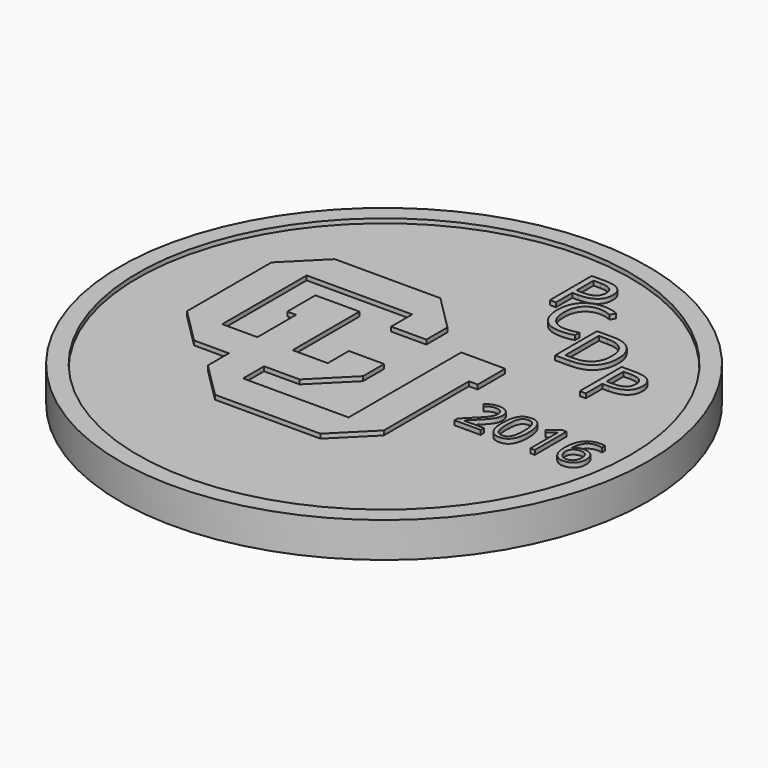
from build123d import *

# Parameters (mm, degrees)
F0_R           = 38.1
F1_DEPTH       = 3.81
F2_R           = 38.1
F2_R_2         = 35.56
F2_TEXT_SIZE   = 10.5833333333
F2_TEXT_SIZE_2 = 8.024699837
F3_DEPTH       = 0.635
F4_R           = 38.1
F4_R_2         = 35.56
F4_TEXT_SIZE   = 14.9135865892
F4_TEXT_SIZE_2 = 16.7777839427
F5_DEPTH       = 0.635


# Not quite as in the source:
# - Text() gives the source's letters only with a copy of the font that has no kerning and outlines rounded to 1/6400 em; it was checked with that copy


with BuildPart() as f1:
    # F0 (on Top) → F1 (new body)
    with BuildSketch(Plane.XY):
        Circle(F0_R)
    extrude(amount=F1_DEPTH)

    # F2 (on face) → F3 (join)
    with BuildSketch(Plane.XY.offset(3.81)):
        Circle(F2_R)
        Circle(F2_R_2, mode=Mode.SUBTRACT)
        Polygon((0, -3.81), (0, 0), (-5.08, 0), (-5.08, -3.81), (-10.16, -3.81), (-10.16, 8.252271885), (-16.51, 8.252271885), (-16.51, 3.172271885), (-15.24, 3.172271885), (-15.24, -3.81), (-20.32, -3.81), (-20.32, 11.43), (-5.08, 11.43), (-5.08, 7.62), (0, 7.62), (0, 11.43), (-5.08, 16.51), (-20.32, 16.51), (-25.4, 11.43), (-25.4, -3.81), (-20.32, -8.89), (-15.2926174924, -8.89), (-10.2126174924, -8.89), (-5.08, -8.89), align=None)
        Polygon((-10.2126174924, -12.6872351393), (-10.2126174924, -8.89), (-15.2926174924, -8.89), (-15.2926174924, -12.6872351393), (-10.189932771, -17.7672351393), (5.0273825076, -17.7672351393), (10.1073825076, -12.6872351393), (10.1073825076, 2.6766592637), (11.3773825076, 2.6766592637), (11.3773825076, 7.6327648607), (5.0273825076, 7.6327648607), (5.0273825076, -12.6872351393), align=None)
        with Locations((12.7, 13.6880021256)):
            Text('D', F2_TEXT_SIZE, font='Open Sans', text_align=(TextAlign.LEFT, TextAlign.BOTTOM))
        with Locations((3.81, 23.8480021256)):
            Text('P', F2_TEXT_SIZE, font='Open Sans', text_align=(TextAlign.LEFT, TextAlign.BOTTOM))
        with Locations((20.32, 8.6080021256)):
            Text('P', F2_TEXT_SIZE, font='Open Sans', text_align=(TextAlign.LEFT, TextAlign.BOTTOM))
        with Locations((6.35, 18.7680021256)):
            Text('C', F2_TEXT_SIZE, font='Open Sans', text_align=(TextAlign.LEFT, TextAlign.BOTTOM))
        with Locations((14.3979993973, -5.7777838827)):
            Text('2016', F2_TEXT_SIZE_2, font='Open Sans', text_align=(TextAlign.LEFT, TextAlign.BOTTOM))
    extrude(amount=F3_DEPTH)

    # F4 (on face) → F5 (join)
    with BuildSketch(Plane(origin=(0, 0, 0), x_dir=(1, 0, 0), z_dir=(0, 0, -1))):
        Circle(F4_R)
        Circle(F4_R_2, mode=Mode.SUBTRACT)
        with Locations((-31.9540211494, 4.434507573)):
            Text('Chandler', F4_TEXT_SIZE, font='Open Sans', text_align=(TextAlign.LEFT, TextAlign.BOTTOM))
        with Locations((-21.8852353573, -16.0951577127)):
            Text('Rowe', F4_TEXT_SIZE_2, font='Open Sans', text_align=(TextAlign.LEFT, TextAlign.BOTTOM))
    extrude(amount=F5_DEPTH)


solid = f1.part
